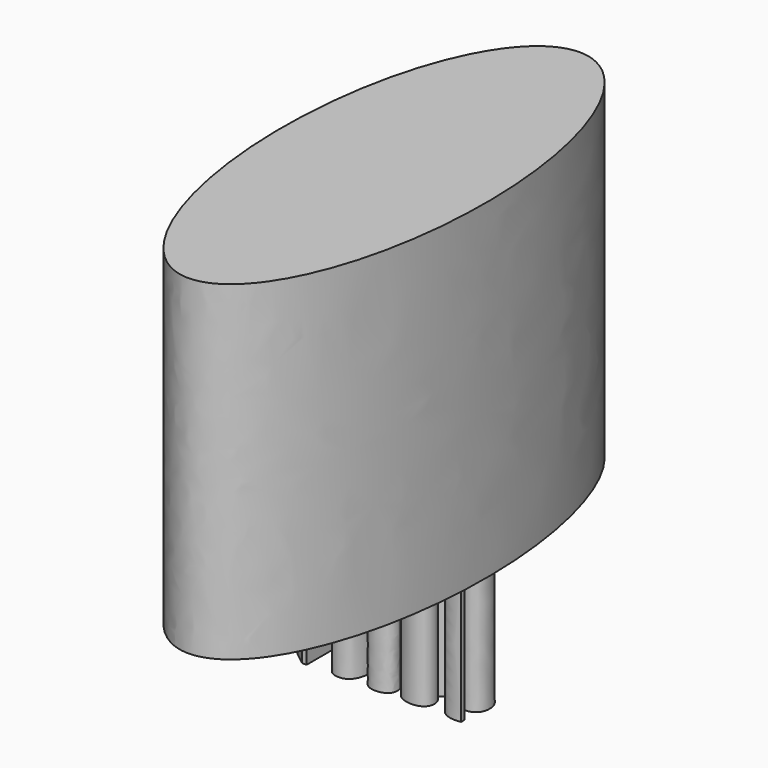
from build123d import *

# Parameters (mm, degrees)
F1_DEPTH     = 116.332
F2_TEXT_SIZE = 22.6169791896
F3_DEPTH     = 47.498


# Not quite as in the source:
# - Text() gives the source's letters only with a copy of the font that has no kerning and outlines rounded to 1/6400 em; it was checked with that copy


with BuildPart() as f1:
    # F0 (on Top) → F1 (new body)
    with BuildSketch(Plane.XY):
        with BuildLine():
            add(Edge.make_bspline(
                [(0, 86.1267894506), (-62.1808675663, 86.1267894506), (-31.0904337832, -43.0633947253), (0, -172.2535789013), (31.0904337832, -43.0633947253), (62.1808675663, 86.1267894506), (0, 86.1267894506)],
                knots=[0, 0, 0, 2.0943951024, 2.0943951024, 4.1887902048, 4.1887902048, 6.2831853072, 6.2831853072, 6.2831853072], degree=2, weights=[1, 0.5, 1, 0.5, 1, 0.5, 1]))
        make_face()
    extrude(amount=-F1_DEPTH)

    # F2 (on face) → F3 (join)
    with BuildSketch(Plane(origin=(0, 0, -116.332), x_dir=(1, 0, 0), z_dir=(0, 0, -1))):
        with Locations((-35.2526130638, -16.2842250165)):
            Text('10836', F2_TEXT_SIZE, font='Open Sans', text_align=(TextAlign.LEFT, TextAlign.BOTTOM))
    extrude(amount=F3_DEPTH)


solid = f1.part
